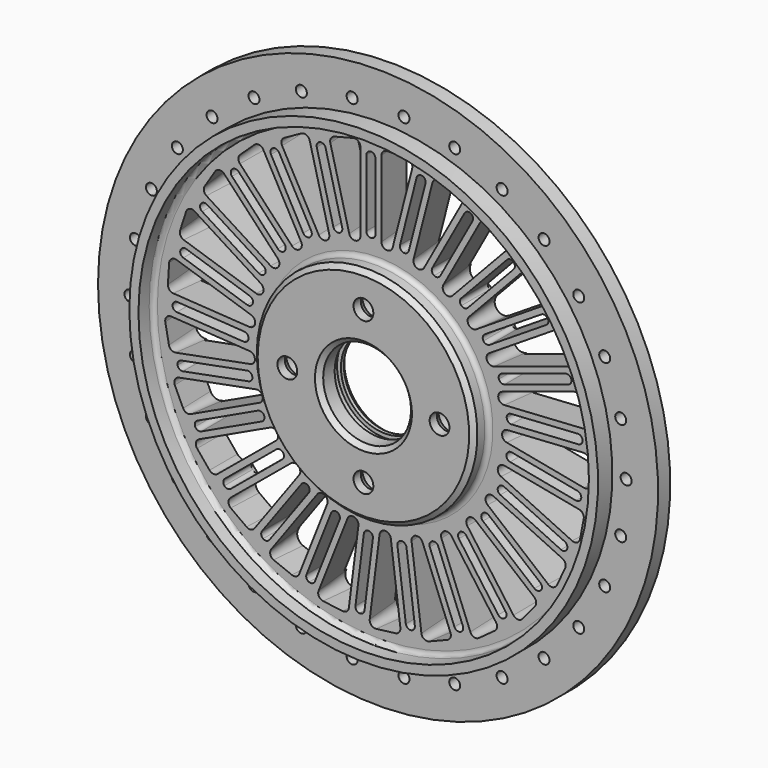
from build123d import *

# Parameters (mm, degrees)
F4_R             = 3.6
F5_DEPTH         = 50
F5_COPIES_COUNT  = 30
F7_COPIES_COUNT  = 4
F8_SIZE          = 3
F9_DEPTH         = 50
F9_TAPER         = 5
F9_COPIES_COUNT  = 25
F10_R            = 135
F10_R_2          = 85
F11_DEPTH        = 3
F13_DEPTH        = 50
F13_COPIES_COUNT = 25


# Not quite as in the source:
# - a pattern or mirror of a feature is missing from the dataset's text; its kind, count and spacing are read off the source's solid


with BuildPart() as f1:
    # F0 (on Top) → F1 (revolve)
    with BuildSketch(Plane.XY):
        with BuildLine():
            ThreePointArc((-75.5, 12), (-73.3786796564, 11.1213203436), (-72.5, 9))
            Line((-72.5, 9), (-72.5, 0))
            Line((-72.5, 0), (-28.85, 0))
            Line((-28.85, 0), (-28.85, 12.4))
            Line((-28.85, 12.4), (-31.45, 12.4))
            Line((-31.45, 12.4), (-31.45, 17.6))
            Line((-31.45, 17.6), (-28.85, 17.6))
            Line((-28.85, 17.6), (-28.85, 20))
            Line((-28.85, 20), (-30, 20))
            ThreePointArc((-30, 20), (-30.7071067812, 20.2928932188), (-31, 21))
            Line((-31, 21), (-31, 23))
            Line((-31, 23), (-67.5, 37))
            Line((-67.5, 37), (-154, 37))
            Line((-154, 37), (-154, 22))
            Line((-154, 22), (-184, 22))
            Line((-184, 22), (-184, 12))
            Line((-184, 12), (-154, 12))
            Line((-154, 12), (-154, 0.2))
            Line((-154, 0.2), (-148, 0.2))
            Line((-148, 0.2), (-148, 9))
            ThreePointArc((-148, 9), (-147.1213203436, 11.1213203436), (-145, 12))
            Line((-145, 12), (-75.5, 12))
        make_face()
    revolve(axis=Axis((0, 8.013517431, 0), (0, -1, 0)))

    # F4 (on Front) → F5 (cut)
    with BuildSketch(Plane.XZ):
        with Locations((163, 0)):
            Circle(F4_R)
    f5 = extrude(amount=-F5_DEPTH, mode=Mode.SUBTRACT)

    # F5_copies: F5 ×30 about axis
    f5_copies_axis = Axis((0, 0, 0), (0, 1, 0))
    for i in range(1, F5_COPIES_COUNT):
        add(f5.rotate(f5_copies_axis, i * 360 / F5_COPIES_COUNT), mode=Mode.SUBTRACT)

    # F6 (on Right) → F7 (revolve, cut)
    with BuildSketch(Plane.YZ):
        Polygon((0, 56.5), (0, 50), (51.0571013514, 50), (51.0571013514, 59), (10.3301270189, 59), (6, 56.5), align=None)
    f7 = revolve(axis=Axis((0, 25.5285506757, 50), (0, 1, 0)), mode=Mode.SUBTRACT)

    # F7_copies: F7 ×4 about axis
    f7_copies_axis = Axis((0, 0, 0), (0, 1, 0))
    for i in range(1, F7_COPIES_COUNT):
        add(f7.rotate(f7_copies_axis, i * 360 / F7_COPIES_COUNT), mode=Mode.SUBTRACT)

    # F8
    f8_edges = [f1.edges().sort_by_distance(p)[0] for p in [
        (72.5, 0, 0),
        (28.85, 0, 0),
    ]]
    chamfer(f8_edges, length=F8_SIZE)

    # F3 (on offset) → F9 (cut)
    with BuildSketch(Plane.XZ.offset(-38)):
        with BuildLine():
            Line((0, 135), (0, 85))
            ThreePointArc((0, 85), (5.2480005986, 79.0473117921), (11.8114989668, 83.507860677))
            Line((11.8114989668, 83.507860677), (24.6493169852, 133.507860677))
            ThreePointArc((24.6493169852, 133.507860677), (23.5787480926, 138.6774423219), (18.8378180184, 141))
            Line((18.8378180184, 141), (6, 141))
            ThreePointArc((6, 141), (1.7573593129, 139.2426406871), (0, 135))
        make_face()
    f9 = extrude(amount=F9_DEPTH, taper=F9_TAPER, mode=Mode.SUBTRACT)

    # F9_copies: F9 ×25 about axis
    f9_copies_axis = Axis((0, 0, 0), (0, 1, 0))
    for i in range(1, F9_COPIES_COUNT):
        add(f9.rotate(f9_copies_axis, i * 360 / F9_COPIES_COUNT), mode=Mode.SUBTRACT)

    # F10 (on offset) → F11 (cut, through all)
    with BuildSketch(Plane.XZ.offset(-38)):
        Circle(F10_R)
        Circle(F10_R_2, mode=Mode.SUBTRACT)
    extrude(amount=F11_DEPTH, mode=Mode.SUBTRACT)

    # F12 (on offset) → F13 (cut)
    with BuildSketch(Plane.XZ.offset(-38)):
        with BuildLine():
            ThreePointArc((-4.7, 135), (-6.8213203436, 134.1213203436), (-7.7, 132))
            Line((-7.7, 132), (-7.7, 88))
            ThreePointArc((-7.7, 88), (-6.8213203436, 85.8786796564), (-4.7, 85))
            ThreePointArc((-4.7, 85), (-2.5786796564, 85.8786796564), (-1.7, 88))
            Line((-1.7, 88), (-1.7, 132))
            ThreePointArc((-1.7, 132), (-2.5786796564, 134.1213203436), (-4.7, 135))
        make_face()
    f13 = extrude(amount=F13_DEPTH, mode=Mode.SUBTRACT)

    # F13_copies: F13 ×25 about axis
    f13_copies_axis = Axis((0, 0, 0), (0, 1, 0))
    for i in range(1, F13_COPIES_COUNT):
        add(f13.rotate(f13_copies_axis, i * 360 / F13_COPIES_COUNT), mode=Mode.SUBTRACT)


solid = f1.part
